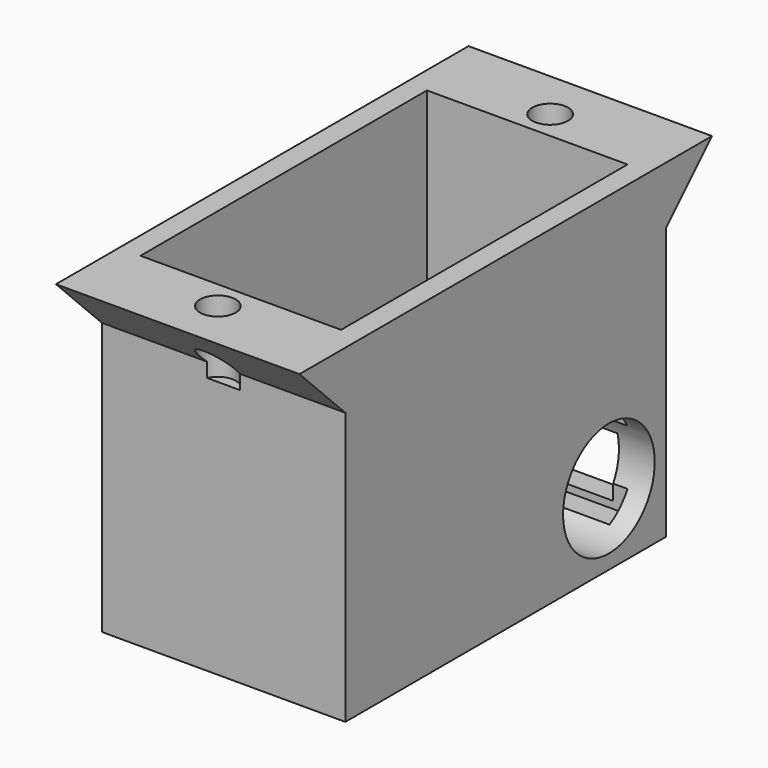
from build123d import *

# Parameters (mm, degrees)
F0_W      = 17
F0_H      = 28
F0_W_2    = 14
F0_H_2    = 25
F1_DEPTH  = 23
F2_DEPTH  = 1.5
F3_W      = 17
F3_H      = 4
F4_DEPTH  = 4
F5_W      = 17
F5_H      = 4
F6_DEPTH  = 4
F5_W_2    = 12
F7_DEPTH  = 1.5
F8_SIZE   = 3.99999
F9_R      = 1.25
F10_DEPTH = 5
F11_R     = 4
F12_DEPTH = 25


# Not quite as in the source:
# - a fillet or chamfer is up to 0.001 mm smaller than in the source, because OpenCascade refuses the exact size


with BuildPart() as f1:
    # F0 (on Top) → F1 (new body)
    with BuildSketch(Plane.XY):
        Rectangle(F0_W, F0_H)
        Rectangle(F0_W_2, F0_H_2, mode=Mode.SUBTRACT)
    extrude(amount=F1_DEPTH)

    # F0 (on Top) → F2 (join)
    with BuildSketch(Plane.XY):
        Rectangle(F0_W_2, F0_H_2)
    extrude(amount=F2_DEPTH)

    # F3 (on face) → F4 (join)
    with BuildSketch(Plane.XZ.offset(14)):
        with Locations((0, 21)):
            Rectangle(F3_W, F3_H)
    extrude(amount=F4_DEPTH)

    # F5 (on face) → F6 (join)
    with BuildSketch(Plane(origin=(0, 14, 0), x_dir=(-1, 0, 0), z_dir=(0, 1, 0))):
        with Locations((0, 21)):
            Rectangle(F5_W, F5_H)
    extrude(amount=F6_DEPTH)

    # F5 (on face) → F7 (cut, through all)
    with BuildSketch(Plane(origin=(0, 14, 0), x_dir=(-1, 0, 0), z_dir=(0, 1, 0))):
        with Locations((0, 4)):
            Rectangle(F5_W_2, F5_H)
    extrude(amount=-F7_DEPTH, mode=Mode.SUBTRACT)

    # F8 (size 4 in the source; OpenCascade refuses exactly that, so slightly less here)
    f8_edges = [f1.edges().sort_by_distance(p)[0] for p in [
        (0, 18, 19),
        (0, -18, 19),
    ]]
    chamfer(f8_edges, length=F8_SIZE)

    # F9 (on face) → F10 (cut)
    with BuildSketch(Plane.XY.offset(23)):
        with Locations((0, 14.5)):
            Circle(F9_R)
        with Locations((0, -14.5)):
            Circle(F9_R)
    extrude(amount=-F10_DEPTH, mode=Mode.SUBTRACT)

    # F11 (on face) → F12 (cut)
    with BuildSketch(Plane(origin=(-8.5, 0, 0), x_dir=(0, -1, 0), z_dir=(-1, 0, 0))):
        with Locations((-9, 5)):
            Circle(F11_R)
    extrude(amount=-F12_DEPTH, mode=Mode.SUBTRACT)


solid = f1.part
